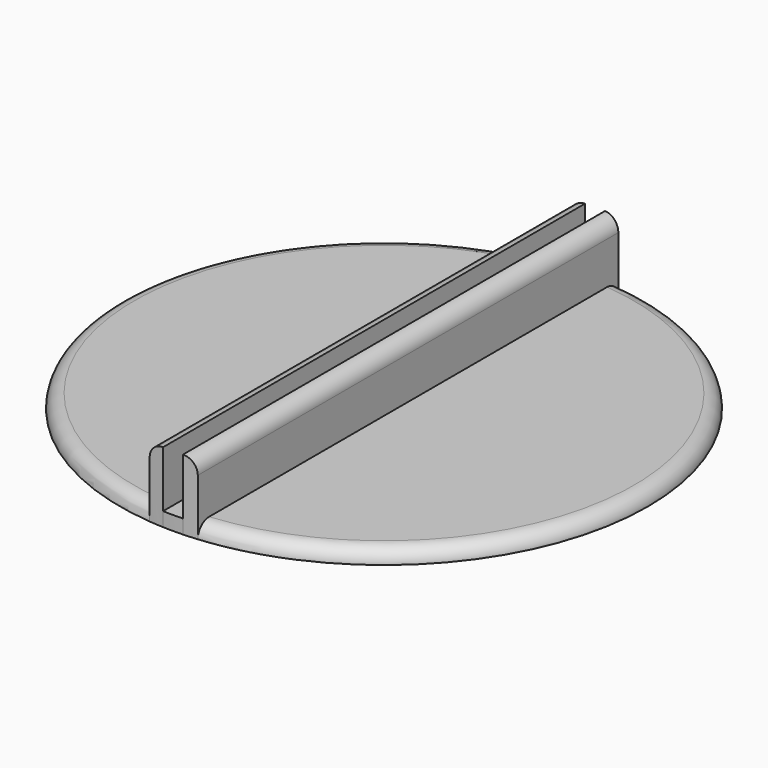
from build123d import *

# Parameters (mm, degrees)
F1_DEPTH      = 1.2
F2_DEPTH      = 6
F3_T2_ANGLE   = 184.8456081764
F3_2_T2_ANGLE = 184.8456081764
F3_3_T1_DEPTH = 50.8128329834
F3_4_T1_DEPTH = 50.8128329834


# Not quite as in the source:
# - a fillet or chamfer that OpenCascade refuses, or shapes differently, is made with other operations: its cross-section is extruded or revolved along the edge and cut away or added


with BuildPart() as f1:
    # F0 (on Top) → F1 (new body)
    with BuildSketch(Plane.XY):
        with BuildLine():
            Line((-2.05, -22.4064164917), (-2.05, 22.4064164917))
            ThreePointArc((-2.05, 22.4064164917), (-22.5, 0), (-2.05, -22.4064164917))
        make_face()
    extrude(amount=F1_DEPTH)

    # F3: fillet of radius 1.2 on 1 edges, made by hand

    # F3_s1 → F3_t2 (revolve, cut)
    with BuildSketch(Plane(origin=(0, 0, 0), x_dir=(0, 0, 1), z_dir=(0.9991060842, -0.0422733077, 0))):
        with BuildLine():
            ThreePointArc((0, -22.5), (0.8485281374, -22.1485281374), (1.2, -21.3))
            Line((1.2, -21.3), (1.2, -22.5))
            Line((1.2, -22.5), (0, -22.5))
        make_face()
    revolve(axis=Axis((0, 0, 1.2), (0, 0, 1)), revolution_arc=F3_T2_ANGLE, mode=Mode.SUBTRACT)


with BuildPart() as f1b:
    # F0 (on Top) → F1, piece 2 (new body)
    with BuildSketch(Plane.XY):
        with BuildLine():
            Line((0.85, -22.4839387119), (0.85, 22.4839387119))
            ThreePointArc((0.85, 22.4839387119), (0, 22.5), (-0.85, 22.4839387119))
            Line((-0.85, 22.4839387119), (-0.85, -22.4839387119))
            ThreePointArc((-0.85, -22.4839387119), (0, -22.5), (0.85, -22.4839387119))
        make_face()
    extrude(amount=F1_DEPTH)


with BuildPart() as f1c:
    # F0 (on Top) → F1, piece 3 (new body)
    with BuildSketch(Plane.XY):
        with BuildLine():
            ThreePointArc((2.05, -22.4064164917), (16.6188898546, -15.1678113121), (22.5, 0))
            ThreePointArc((22.5, 0), (16.6188898546, 15.1678113121), (2.05, 22.4064164917))
            Line((2.05, 22.4064164917), (2.05, -22.4064164917))
        make_face()
    extrude(amount=F1_DEPTH)

    # F3#2: fillet of radius 1.2 on 1 edges, made by hand

    # F3_2_s1 → F3_2_t2 (revolve, cut)
    with BuildSketch(Plane(origin=(0, 0, 0), x_dir=(0, 0, 1), z_dir=(-0.9991060842, -0.0422733077, 0))):
        with BuildLine():
            ThreePointArc((0, 22.5), (0.8485281374, 22.1485281374), (1.2, 21.3))
            Line((1.2, 21.3), (1.2, 22.5))
            Line((1.2, 22.5), (0, 22.5))
        make_face()
    revolve(axis=Axis((0, 0, 1.2), (0, 0, -1)), revolution_arc=F3_2_T2_ANGLE, mode=Mode.SUBTRACT)


with BuildPart() as f2:
    # F0 (on Top) → F2 (new body)
    with BuildSketch(Plane.XY):
        with BuildLine():
            Line((2.05, -22.4064164917), (2.05, 22.4064164917))
            ThreePointArc((2.05, 22.4064164917), (1.4505179846, 22.4531957097), (0.85, 22.4839387119))
            Line((0.85, 22.4839387119), (0.85, -22.4839387119))
            ThreePointArc((0.85, -22.4839387119), (1.4505179846, -22.4531957097), (2.05, -22.4064164917))
        make_face()
    extrude(amount=F2_DEPTH)

    # F3#3: fillet of radius 1.2 on 1 edges, made by hand

    # F3_3_s2 → F3_3_t1 (cut)
    with BuildSketch(Plane.XZ.offset(-25.4064164917)):
        with BuildLine():
            ThreePointArc((2.05, 4.8), (1.6985281374, 5.6485281374), (0.85, 6))
            Line((0.85, 6), (2.05, 6))
            Line((2.05, 6), (2.05, 4.8))
        make_face()
    extrude(amount=F3_3_T1_DEPTH, mode=Mode.SUBTRACT)


with BuildPart() as f2b:
    # F0 (on Top) → F2, piece 2 (new body)
    with BuildSketch(Plane.XY):
        with BuildLine():
            Line((-0.85, -22.4839387119), (-0.85, 22.4839387119))
            ThreePointArc((-0.85, 22.4839387119), (-1.4505179846, 22.4531957097), (-2.05, 22.4064164917))
            Line((-2.05, 22.4064164917), (-2.05, -22.4064164917))
            ThreePointArc((-2.05, -22.4064164917), (-1.4505179846, -22.4531957097), (-0.85, -22.4839387119))
        make_face()
    extrude(amount=F2_DEPTH)

    # F3#4: fillet of radius 1.2 on 1 edges, made by hand

    # F3_4_s2 → F3_4_t1 (cut)
    with BuildSketch(Plane.XZ.offset(-25.4064164917)):
        with BuildLine():
            ThreePointArc((-2.05, 4.8), (-1.6985281374, 5.6485281374), (-0.85, 6))
            Line((-0.85, 6), (-2.05, 6))
            Line((-2.05, 6), (-2.05, 4.8))
        make_face()
    extrude(amount=F3_4_T1_DEPTH, mode=Mode.SUBTRACT)


solid = Compound([f1.part, f1b.part, f1c.part, f2.part, f2b.part])
